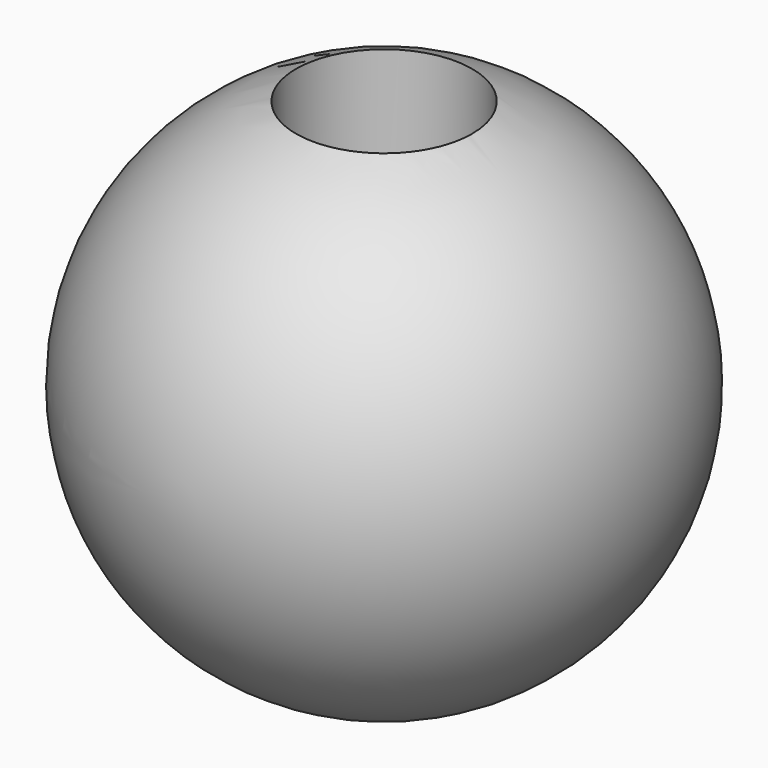
from build123d import *

# Parameters (mm, degrees)
F4_R     = 3.175
F5_DEPTH = 9.525


# Not quite as in the source:
# - a length typed as a fraction of an inch, garbled in the dataset ("3 / 203.2 mm" for 3/8 in), is restored


with BuildPart() as f2:
    # F1 (on Top) → F2 (revolve)
    with BuildSketch(Plane.XY):
        with BuildLine():
            Line((0, -9.525), (0, 9.525))
            ThreePointArc((0, 9.525), (-9.525, 0), (0, -9.525))
        make_face()
    revolve(axis=Axis((0, 0, 0), (0, -1, 0)))

    # F4 (on offset) → F5 (cut)
    with BuildSketch(Plane.XY.offset(9.525)):
        Circle(F4_R)
    extrude(amount=-F5_DEPTH, mode=Mode.SUBTRACT)


solid = f2.part
